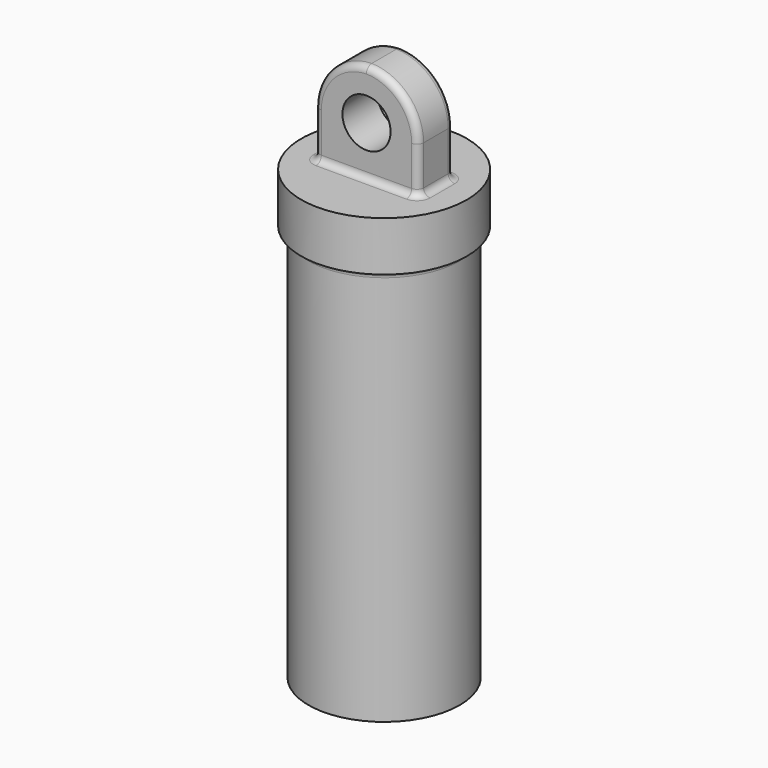
from build123d import *

# Parameters (mm, degrees)
F0_R        = 28.9544209137
F0_R_2      = 21.0693
F1_DEPTH    = 152.4
F2_R        = 31.75
F3_DEPTH    = 19.05
F4_W        = 39.7148355842
F4_H        = 16.8466605246
F5_DEPTH    = 38.1
F6_R        = 9.2348971927
F7_DEPTH    = 25.4
F8_T1_DEPTH = 118.4466605246
F9_R        = 2.54


# Not quite as in the source:
# - a fillet or chamfer that OpenCascade refuses, or shapes differently, is made with other operations: its cross-section is extruded or revolved along the edge and cut away or added


with BuildPart() as f1:
    # F0 (on Top) → F1 (new body)
    with BuildSketch(Plane.XY):
        Circle(F0_R)
        Circle(F0_R_2, mode=Mode.SUBTRACT)
    extrude(amount=F1_DEPTH)

    # F2 (on face) → F3 (join)
    with BuildSketch(Plane.XY.offset(152.4)):
        Circle(F2_R)
    extrude(amount=F3_DEPTH)

    # F4 (on face) → F5 (join)
    with BuildSketch(Plane.XY.offset(171.45)):
        Rectangle(F4_W, F4_H)
    extrude(amount=F5_DEPTH)

    # F6 (on face) → F7 (cut)
    with BuildSketch(Plane.XZ.offset(8.4233302623)):
        with Locations((0, 190.5)):
            Circle(F6_R)
    extrude(amount=-F7_DEPTH, mode=Mode.SUBTRACT)

    # F8: fillet of radius 20.32 on 2 edges, made by hand

    # F8_s2 → F8_t1 (cut)
    with BuildSketch(Plane.XZ.offset(-59.2233302623)):
        with BuildLine():
            ThreePointArc((19.8574177921, 189.23), (13.9058275858, 203.5984097937), (-0.4625822079, 209.55))
            Line((-0.4625822079, 209.55), (19.8574177921, 209.55))
            Line((19.8574177921, 209.55), (19.8574177921, 189.23))
        make_face()
        with BuildLine():
            ThreePointArc((-19.8574177921, 189.23), (-13.9058275858, 203.5984097937), (0.4625822079, 209.55))
            Line((0.4625822079, 209.55), (-19.8574177921, 209.55))
            Line((-19.8574177921, 209.55), (-19.8574177921, 189.23))
        make_face()
    extrude(amount=F8_T1_DEPTH, mode=Mode.SUBTRACT)

    # F9
    f9_edges = [f1.edges().sort_by_distance(p)[0] for p in [
        (19.857418, -8.42333, 180.34),
        (14.068455, -8.42333, 203.433921),
        (-14.068455, -8.42333, 203.433921),
        (-19.857418, -8.42333, 180.34),
        (0, -8.42333, 171.45),
        (19.857418, 0, 171.45),
        (-28.954421, 0, 152.4),
        (-21.0693, 0, 152.4),
        (19.857418, 8.42333, 180.34),
        (14.068455, 8.42333, 203.433921),
        (-14.068455, 8.42333, 203.433921),
        (0, 8.42333, 171.45),
        (-19.857418, 0, 171.45),
        (-19.857418, 8.42333, 180.34),
    ]]
    fillet(f9_edges, radius=F9_R)


solid = f1.part
